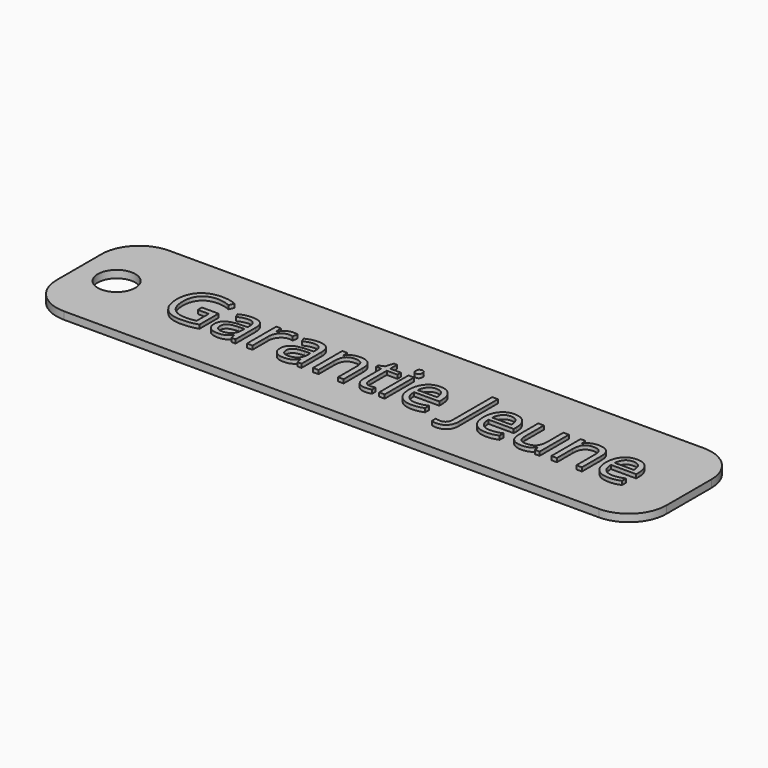
from build123d import *

# Parameters (mm, degrees)
F0_W         = 65
F0_H         = 14
F0_R         = 2
F1_DEPTH     = 0.8
F2_R         = 4
F3_TEXT_SIZE = 7.2956089554
F4_DEPTH     = 0.4


# Not quite as in the source:
# - a feature names something its author has since deleted; it is built from what else it names
# - Text() gives the source's letters only with a copy of the font that has no kerning and outlines rounded to 1/6400 em; it was checked with that copy


with BuildPart() as f1:
    # F0 (on Top) → F1 (new body)
    with BuildSketch(Plane.XY):
        with Locations((32.5, 0)):
            Rectangle(F0_W, F0_H)
        with Locations((4, 0)):
            Circle(F0_R, mode=Mode.SUBTRACT)
    extrude(amount=F1_DEPTH)

    # F2
    f2_edges = [f1.edges().sort_by_distance(p)[0] for p in [
        (0, -7, 0.4),
        (65, -7, 0.4),
        (65, 7, 0.4),
        (0, 7, 0.4),
    ]]
    fillet(f2_edges, radius=F2_R)

    # F3 (on face) → F4 (join)
    with BuildSketch(Plane.XY.offset(0.8)):
        with Locations((10, -2.6264192239)):
            Text('Garantie Jeune', F3_TEXT_SIZE, font='Open Sans', text_align=(TextAlign.LEFT, TextAlign.BOTTOM))
    extrude(amount=F4_DEPTH)


solid = f1.part
